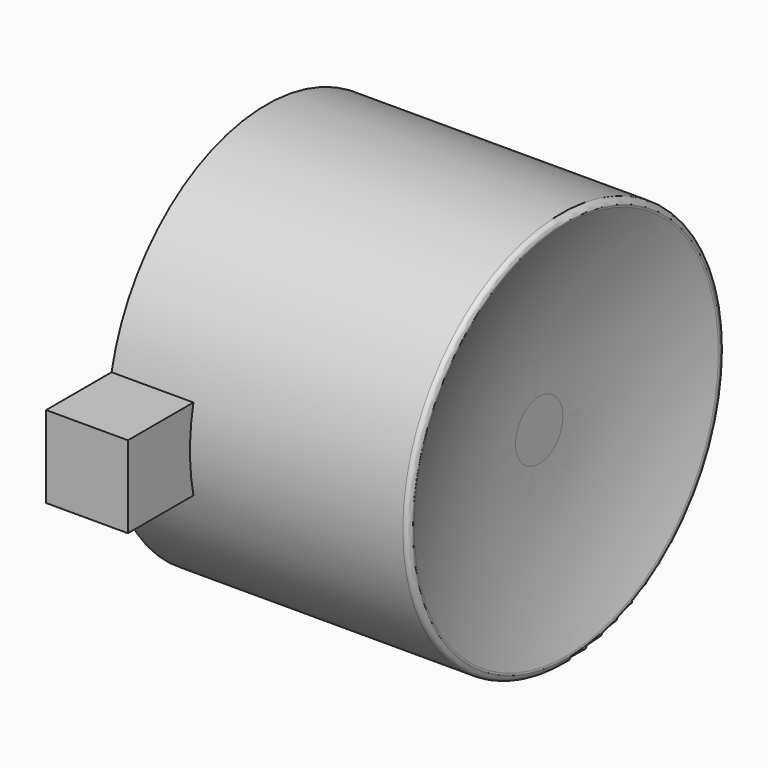
from build123d import *

# Parameters (mm, degrees)
F0_R     = 3.625
F1_DEPTH = 2.75
F3_DEPTH = 1.5
F4_R     = 3.5
F5_DEPTH = 0.5
F7_R     = 0.1


# Not quite as in the source:
# - a fillet or chamfer that OpenCascade refuses, or shapes differently, is made with other operations: its cross-section is extruded or revolved along the edge and cut away or added


with BuildPart() as f1:
    # F0 (on Right) → F1 (new body, symmetric)
    with BuildSketch(Plane.YZ):
        Circle(F0_R)
    extrude(amount=F1_DEPTH, both=True)

    # F2 (on face) → F3 (join)
    with BuildSketch(Plane(origin=(-2.75, 0, 0), x_dir=(0, -1, 0), z_dir=(-1, 0, 0))):
        with BuildLine():
            Line((3.5465652398, -0.75), (5.0465652398, -0.75))
            Line((5.0465652398, -0.75), (5.0465652398, 0.75))
            Line((5.0465652398, 0.75), (3.5465652398, 0.75))
            ThreePointArc((3.5465652398, 0.75), (3.625, 0), (3.5465652398, -0.75))
        make_face()
        with BuildLine():
            Line((-3.5465652398, 0.75), (-5.0465652398, 0.75))
            Line((-5.0465652398, 0.75), (-5.0465652398, -0.75))
            Line((-5.0465652398, -0.75), (-3.5465652398, -0.75))
            ThreePointArc((-3.5465652398, -0.75), (-3.625, 0), (-3.5465652398, 0.75))
        make_face()
    extrude(amount=-F3_DEPTH)

    # F4 (on face) → F5 (cut)
    with BuildSketch(Plane.YZ.offset(2.75)):
        Circle(F4_R)
    extrude(amount=-F5_DEPTH, mode=Mode.SUBTRACT)

    # F6: fillet of radius 9 on 1 edges, made by hand

    # F6_s1 → F6_t2 (revolve)
    with BuildSketch(Plane.XY):
        with BuildLine():
            ThreePointArc((2.75, 3.5), (2.3758803254, 2.0419601084), (2.25, 0.5419601084))
            Line((2.25, 0.5419601084), (2.25, 3.5))
            Line((2.25, 3.5), (2.75, 3.5))
        make_face()
    revolve(axis=Axis((2.25, 0, 0), (1, 0, 0)))

    # F7
    f7_edges = [f1.edges().sort_by_distance(p)[0] for p in [
        (2.75, -3.5, 0),
        (2.75, -3.625, 0),
    ]]
    fillet(f7_edges, radius=F7_R)


solid = f1.part
